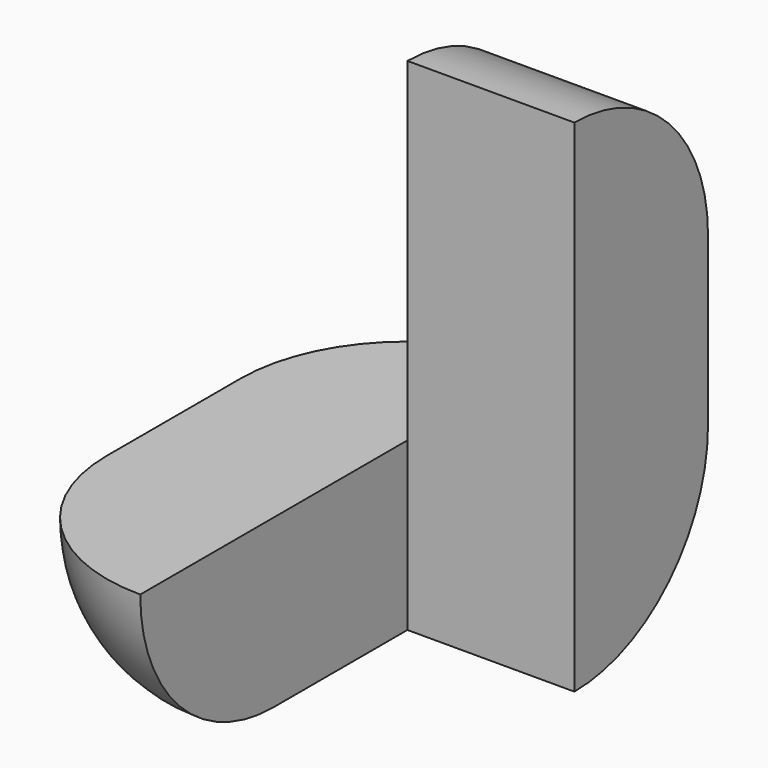
from build123d import *

# Parameters (mm, degrees)
F1_DEPTH = 25.4
F2_W     = 25.4
F2_H     = 25.4
F3_DEPTH = 50.8
F4_R     = 25.39999


# Not quite as in the source:
# - a fillet or chamfer is up to 0.001 mm smaller than in the source, because OpenCascade refuses the exact size


with BuildPart() as f1:
    # F0 (on Top) → F1 (new body)
    with BuildSketch(Plane.XY):
        Polygon((0, 76.2), (0, 0), (25.4, 0), (25.4, 50.8), (50.8, 50.8), (50.8, 76.2), align=None)
    extrude(amount=F1_DEPTH)

    # F2 (on face) → F3 (join)
    with BuildSketch(Plane.XY.offset(25.4)):
        with Locations((38.1, 63.5)):
            Rectangle(F2_W, F2_H)
    extrude(amount=F3_DEPTH)

    # F4 (radius 25.4 in the source; OpenCascade refuses exactly that, so slightly less here)
    f4_edges = [f1.edges().sort_by_distance(p)[0] for p in [
        (0, 38.1, 0),
        (0, 0, 12.7),
        (0, 76.2, 12.7),
        (25.4, 76.2, 0),
        (38.1, 76.2, 76.2),
        (12.7, 0, 0),
    ]]
    fillet(f4_edges, radius=F4_R)


solid = f1.part
